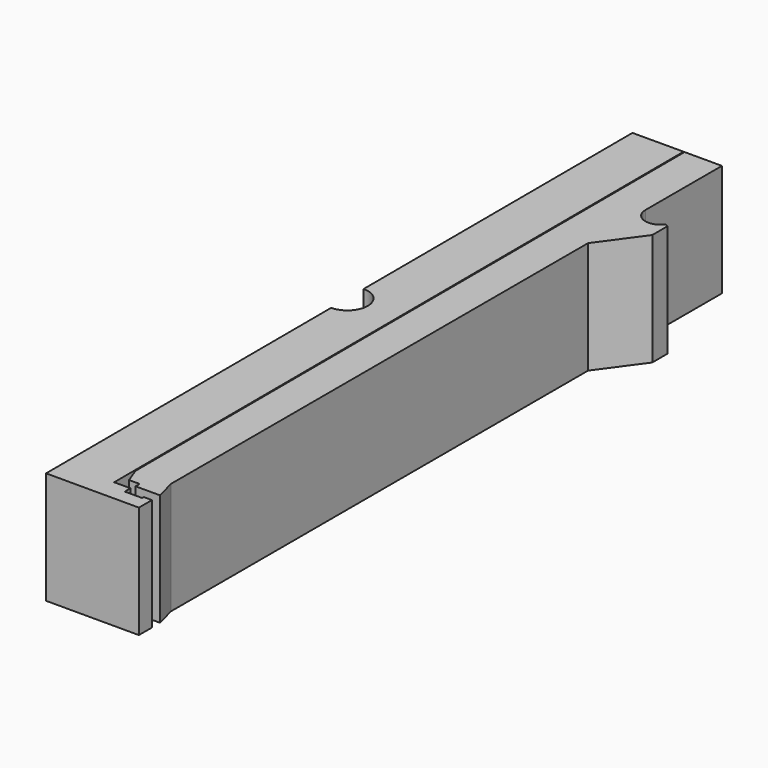
from build123d import *

# Parameters (mm, degrees)
F1_DEPTH = 11
F2_W     = 4
F2_H     = 4
F3_REACH = 77.7696273196
F4_W     = 3.9
F4_H     = 3.9
F5_DEPTH = 67.39
F6_R     = 2
F7_DEPTH = 25
F9_DEPTH = 11


with BuildPart() as f1:
    # F0 (on Top) → F1 (new body)
    with BuildSketch(Plane.XY):
        Polygon((-25.8345385283, -6.3107501626), (-25.8345385283, -4.7107501626), (-26.6345385283, -4.7107501626), (-26.6345385283, -4.9107501626), (-28.3345385283, -4.9107501626), (-28.3345385283, -4.7107501626), (-28.3345385283, -4.2107501626), (-29.9345385283, -4.2107501626), (-30.1356901966, 65.7889608226), (-35.1356695527, 65.7745928463), (-34.9285245974, -6.3107501626), (-31.0404077172, -6.3107501626), align=None)
    extrude(amount=F1_DEPTH)

    f3_end = Plane(origin=(-29.1345385283, -4.2107501626, 5.5), x_dir=(0, 0, 1), z_dir=(0, 1, 0))
    # F2 (on face) → F3 (cut, up to a plane its end follows)
    with BuildSketch(Plane(origin=(-0.1892989125, 65.875014986, 0), x_dir=(-0.9999958712, -0.0028735953, 0), z_dir=(-0.0028735953, 0.9999958712, 0))):
        with Locations((29.9465149268, 5.5)):
            Rectangle(F2_W, F2_H)
    f3_long = extrude(amount=-F3_REACH, mode=Mode.PRIVATE)
    add(split(f3_long, bisect_by=f3_end, keep=Keep.TOP, mode=Mode.PRIVATE), mode=Mode.SUBTRACT)

    # F6 (on face) → F7 (cut)
    with BuildSketch(Plane.XY.offset(11)):
        with Locations((-35.0349817941, 30.7357882368)):
            Circle(F6_R)
    extrude(amount=-F7_DEPTH, mode=Mode.SUBTRACT)


with BuildPart() as f1b:
    # F0 (on Top) → F1, piece 2 (new body)
    with BuildSketch(Plane.XY):
        Polygon((-28.2345385283, -3.7107501626), (-25.8400786679, -3.7107501626), (-26.3759770527, -1.7107501626), (-26.3759770527, 65.7889608226), (-30.0356901966, 65.7889608226), (-29.8417225461, -1.7107501626), (-29.281405732, -3.2107501626), (-28.2345385283, -3.2107501626), align=None)
    extrude(amount=F1_DEPTH)

    # F4 (on face) → F5 (join)
    with BuildSketch(Plane(origin=(0, 65.7889608226, 0), x_dir=(-1, 0, 0), z_dir=(0, 1, 0))):
        with Locations((30.0356901966, 5.5)):
            Rectangle(F4_W, F4_H)
    extrude(amount=-F5_DEPTH)

    # F8 (on face) → F9 (join, through all)
    with BuildSketch(Plane.XY.offset(11)):
        with BuildLine():
            ThreePointArc((-23.6712550626, 55.5191615881), (-25.3465708344, 54.9885621917), (-26.3759770527, 56.4128309488))
            Line((-26.3759770527, 56.4128309488), (-26.3759770527, 49.3795908988))
            Line((-26.3759770527, 49.3795908988), (-23.3791565106, 53.5104437786))
            Line((-23.3791565106, 53.5104437786), (-23.3791565106, 55.3792828116))
            Line((-23.3791565106, 55.3792828116), (-23.6712550626, 55.5191615881))
        make_face()
    extrude(amount=-F9_DEPTH)


solid = Compound([f1.part, f1b.part])
